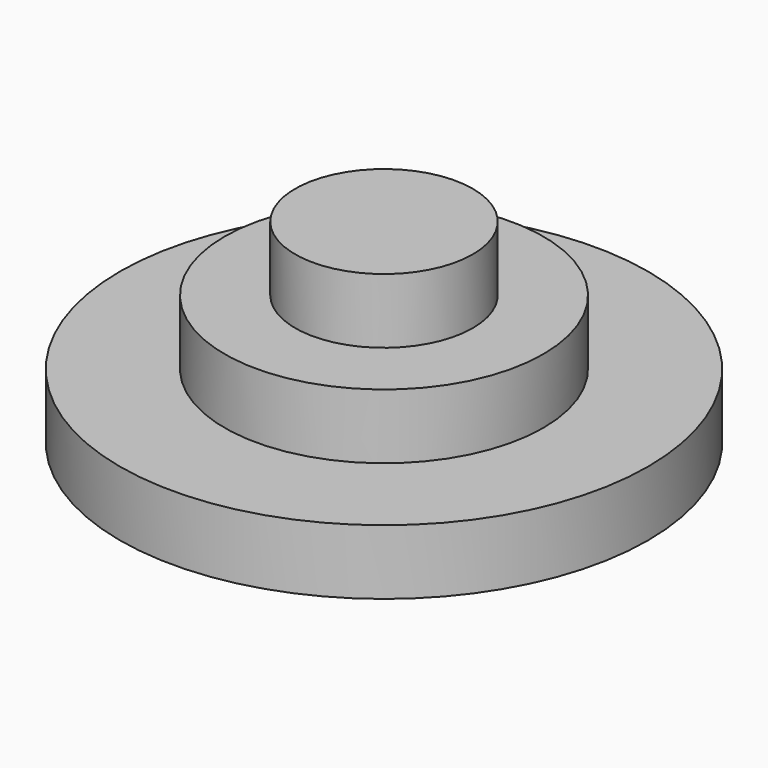
from build123d import *

# Parameters (mm, degrees)
F0_R     = 3.8227
F1_DEPTH = 2.794
F0_R_2   = 6.858
F2_DEPTH = 2.794
F3_R     = 11.3665
F3_R_2   = 6.858
F4_DEPTH = 2.794


with BuildPart() as f1:
    # F0 (on Top) → F1 (new body)
    with BuildSketch(Plane.XY):
        Circle(F0_R)
    extrude(amount=F1_DEPTH)

    # F0 (on Top) → F2 (join)
    with BuildSketch(Plane.XY):
        Circle(F0_R_2)
        Circle(F0_R, mode=Mode.SUBTRACT)
        Circle(F0_R)
    extrude(amount=-F2_DEPTH)

    # F3 (on face) → F4 (join)
    with BuildSketch(Plane(origin=(0, 0, -2.794), x_dir=(1, 0, 0), z_dir=(0, 0, -1))):
        Circle(F3_R)
        Circle(F3_R_2, mode=Mode.SUBTRACT)
        Circle(F3_R_2)
    extrude(amount=F4_DEPTH)


solid = f1.part
